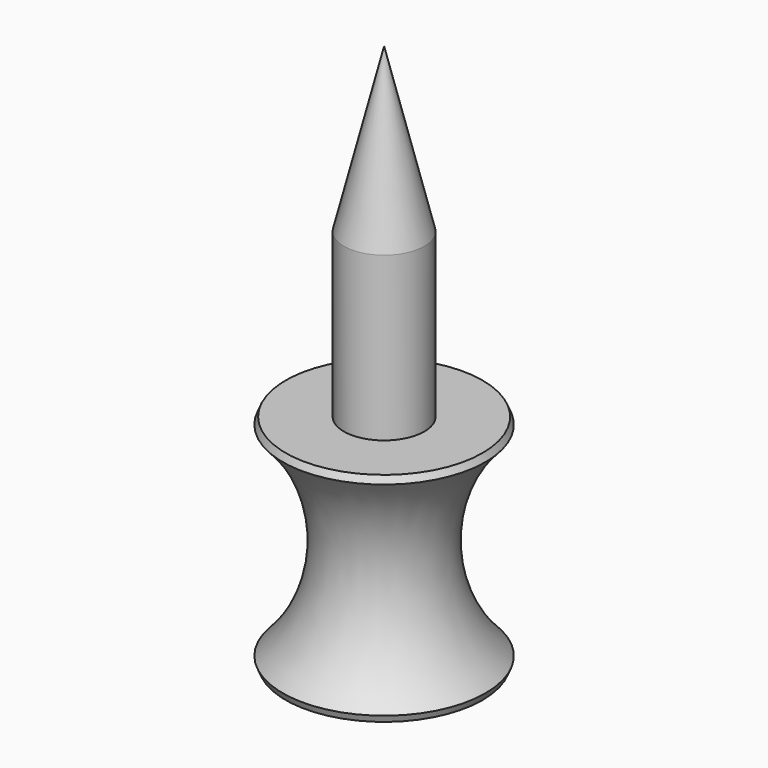
from build123d import *


# Not quite as in the source:
# - a fillet or chamfer that OpenCascade refuses, or shapes differently, is made with other operations: its cross-section is extruded or revolved along the edge and cut away or added


with BuildPart() as f1:
    # F0 (on Front) → F1 (revolve)
    with BuildSketch(Plane.XZ):
        with BuildLine():
            Line((0, 31.75), (0, 6.35))
            Line((0, 6.35), (4.7625, 0))
            Line((4.7625, 0), (6.35, 0))
            ThreePointArc((6.35, 0), (3.4925, 6.35), (6.35, 12.7))
            Line((6.35, 12.7), (2.3495, 12.7))
            Line((2.3495, 12.7), (2.3495, 22.225))
            Line((2.3495, 22.225), (0, 31.75))
        make_face()
    revolve(axis=Axis((0, 0, 19.05), (0, 0, -1)))

    # F2: chamfer of 0.635 on 2 edges, made by hand

    # F2_s1 → F2_t2 (revolve, cut)
    with BuildSketch(Plane.XZ):
        with BuildLine():
            Line((5.929083675, 12.2670736629), (5.7374458679, 12.7234188432))
            Line((5.7374458679, 12.7234188432), (5.7374458679, 12.7361188432))
            ThreePointArc((5.7374458679, 12.7361188432), (6.043722934, 12.7127), (6.35, 12.7127))
            Line((6.35, 12.7127), (6.3584226611, 12.6904948025))
            ThreePointArc((6.3584226611, 12.6904948025), (6.1365228233, 12.4867090771), (5.9381511191, 12.2581814496))
            Line((5.9381511191, 12.2581814496), (5.929083675, 12.2670736629))
        make_face()
    revolve(axis=Axis((0, 0, 12.7), (0, 0, -1)), mode=Mode.SUBTRACT)

    # F2_s3 → F2_t4 (revolve, cut)
    with BuildSketch(Plane.XZ):
        with BuildLine():
            Line((5.7374458679, -0.0234188432), (5.929083675, 0.4329263371))
            Line((5.929083675, 0.4329263371), (5.9381511191, 0.4418185504))
            ThreePointArc((5.9381511191, 0.4418185504), (6.1365228233, 0.2132909229), (6.3584226611, 0.0095051975))
            Line((6.3584226611, 0.0095051975), (6.35, -0.0127))
            ThreePointArc((6.35, -0.0127), (6.043722934, -0.0127), (5.7374458679, -0.0361188432))
            Line((5.7374458679, -0.0361188432), (5.7374458679, -0.0234188432))
        make_face()
    revolve(axis=Axis((0, 0, 0), (0, 0, -1)), mode=Mode.SUBTRACT)


solid = f1.part
